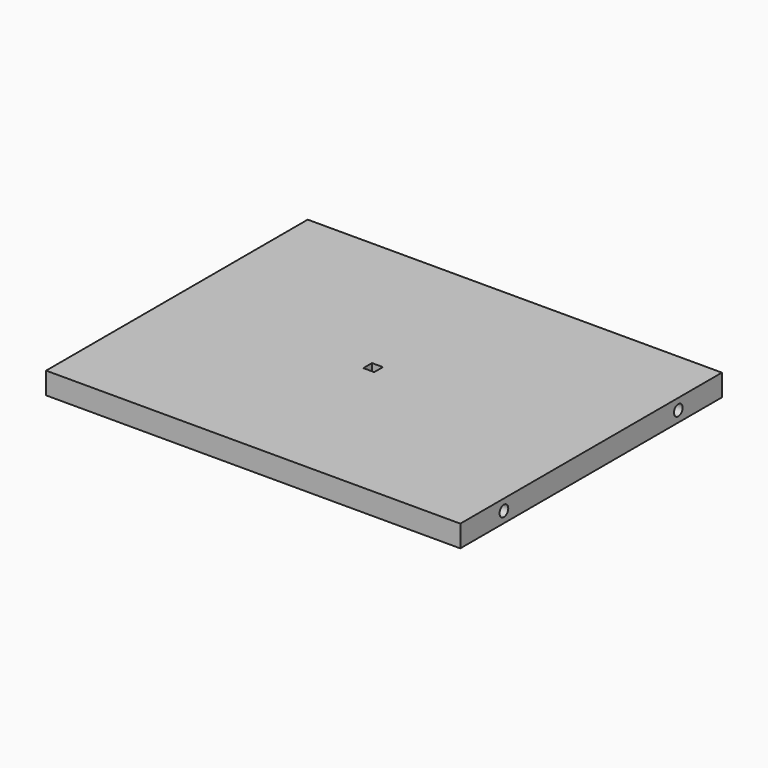
from build123d import *

# Parameters (mm, degrees)
F0_W     = 150
F0_H     = 150
F0_W_2   = 5
F0_H_2   = 5
F1_DEPTH = 10
F3_R     = 2.5
F4_DEPTH = 25
F5_W     = 150
F5_H     = 10
F5_R     = 2.5
F6_DEPTH = 15


# Not quite as in the source:
# - a feature of the source that left no trace in its solid (it failed there, or was rolled back) is left out


with BuildPart() as f1:
    # F0 (on Top) → F1 (new body)
    with BuildSketch(Plane.XY):
        Rectangle(F0_W, F0_H)
        Rectangle(F0_W_2, F0_H_2, mode=Mode.SUBTRACT)
    extrude(amount=F1_DEPTH)

    # F3 (on face) → F4 (join)
    with BuildSketch(Plane.YZ.offset(75)):
        Polygon((75, 0), (75, 10), (-75, 10), (-75, 0), (0, 0), align=None)
        with Locations((-50, 5)):
            Circle(F3_R, mode=Mode.SUBTRACT)
        with Locations((50, 5)):
            Circle(F3_R, mode=Mode.SUBTRACT)
    extrude(amount=F4_DEPTH)

    # F5 (on face) → F6 (join)
    with BuildSketch(Plane(origin=(-75, 0, 0), x_dir=(0, -1, 0), z_dir=(-1, 0, 0))):
        with Locations((0, 5)):
            Rectangle(F5_W, F5_H)
        with Locations((-50, 5)):
            Circle(F5_R, mode=Mode.SUBTRACT)
        with Locations((50, 5)):
            Circle(F5_R, mode=Mode.SUBTRACT)
    extrude(amount=F6_DEPTH)


solid = f1.part
